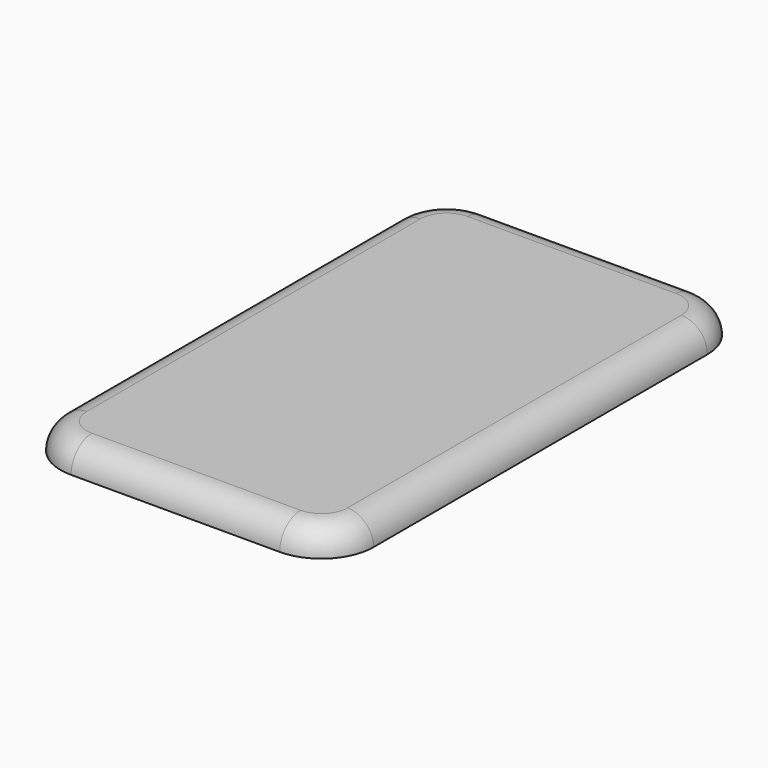
from build123d import *

# Parameters (mm, degrees)
F1_DEPTH = 10
F2_R     = 9.99999


# Not quite as in the source:
# - a fillet or chamfer is up to 0.001 mm smaller than in the source, because OpenCascade refuses the exact size


with BuildPart() as f1:
    # F0 (on Top) → F1 (new body)
    with BuildSketch(Plane.XY):
        with BuildLine():
            Line((40, 100), (-40, 100))
            ThreePointArc((-40, 100), (-54.1421356237, 94.1421356237), (-60, 80))
            Line((-60, 80), (-60, -80))
            ThreePointArc((-60, -80), (-54.1421356237, -94.1421356237), (-40, -100))
            Line((-40, -100), (40, -100))
            ThreePointArc((40, -100), (54.1421356237, -94.1421356237), (60, -80))
            Line((60, -80), (60, 80))
            ThreePointArc((60, 80), (54.1421356237, 94.1421356237), (40, 100))
        make_face()
    extrude(amount=F1_DEPTH)

    # F2 (radius 10 in the source; OpenCascade refuses exactly that, so slightly less here)
    f2_edges = [f1.edges().sort_by_distance(p)[0] for p in [
        (-60, 0, 10),
    ]]
    fillet(f2_edges, radius=F2_R)


solid = f1.part
